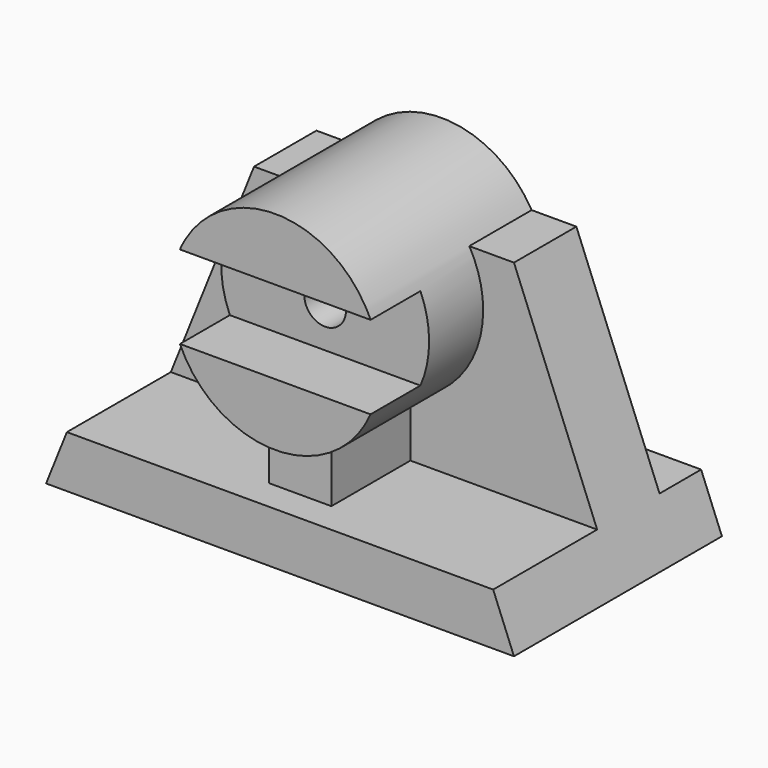
from build123d import *

# Parameters (mm, degrees)
F0_W      = 90
F0_H      = 50
F1_DEPTH  = 10
F2_W      = 90
F2_H      = 15
F3_DEPTH  = 40
F4_SIZE2  = 49.99999
F4_SIZE   = 19.99999
F5_SIZE2  = 19.99999
F5_SIZE   = 49.99999
F7_DEPTH  = 25
F8_DEPTH  = 15
F9_DEPTH  = 13
F10_DEPTH = 19
F11_R     = 4
F12_DEPTH = 40


# Not quite as in the source:
# - a fillet or chamfer is up to 0.001 mm smaller than in the source, because OpenCascade refuses the exact size


with BuildPart() as f1:
    # F0 (on Top) → F1 (new body)
    with BuildSketch(Plane.XY):
        with Locations((0.9217737243, 10.8652876893)):
            Rectangle(F0_W, F0_H)
    extrude(amount=F1_DEPTH)

    # F2 (on face) → F3 (join)
    with BuildSketch(Plane.XY.offset(10)):
        with Locations((0.9217737243, 18.3652876893)):
            Rectangle(F2_W, F2_H)
    extrude(amount=F3_DEPTH)

    # F4 (size 20 and 50 in the source; OpenCascade refuses exactly that, so slightly less here)
    f4_edges = [f1.edges().sort_by_distance(p)[0] for p in [
        (-44.078226, 18.365288, 50),
    ]]
    f4_side = f1.faces().sort_by_distance((0.921774, 18.365288, 50))[0]
    chamfer(f4_edges, length=F4_SIZE, length2=F4_SIZE2, reference=f4_side)

    # F5 (size 50 and 20 in the source; OpenCascade refuses exactly that, so slightly less here)
    f5_edges = [f1.edges().sort_by_distance(p)[0] for p in [
        (45.921774, 18.365288, 50),
    ]]
    f5_side = f1.faces().sort_by_distance((45.921774, 14.956197, 18.636364))[0]
    chamfer(f5_edges, length=F5_SIZE, length2=F5_SIZE2, reference=f5_side)

    # F6 (on face) → F7 (join)
    with BuildSketch(Plane.XZ.offset(-10.8652876893)):
        with BuildLine():
            Line((-17.3205080757, 50), (17.3205080757, 50))
            ThreePointArc((17.3205080757, 50), (0, 60), (-17.3205080757, 50))
        make_face()
        with BuildLine():
            Line((-18.3303027798, 48), (18.3303027798, 48))
            ThreePointArc((18.3303027798, 48), (17.8534332458, 49.0141511711), (17.3205080757, 50))
            Line((17.3205080757, 50), (-17.3205080757, 50))
            ThreePointArc((-17.3205080757, 50), (-17.8534332458, 49.0141511711), (-18.3303027798, 48))
        make_face()
        with BuildLine():
            ThreePointArc((6, 20.9212159717), (13.3669657075, 25.1230302893), (18.3303027798, 32))
            Line((18.3303027798, 32), (-18.3303027798, 32))
            ThreePointArc((-18.3303027798, 32), (-13.3669657075, 25.1230302893), (-6, 20.9212159717))
            ThreePointArc((-6, 20.9212159717), (0, 20), (6, 20.9212159717))
        make_face()
    extrude(amount=F7_DEPTH)

    # F8 (add): a face of the model
    f8_faces = [f1.faces().sort_by_distance(p)[0] for p in [
        (0, 10.8652876893, 54.100403238),
    ]]
    extrude(f8_faces, amount=F8_DEPTH)

    # F6 (on face) → F9 (join)
    with BuildSketch(Plane.XZ.offset(-10.8652876893)):
        with BuildLine():
            ThreePointArc((18.3303027798, 32), (19.5781262586, 35.9138071262), (20, 40))
            ThreePointArc((20, 40), (19.5781262586, 44.0861928738), (18.3303027798, 48))
            Line((18.3303027798, 48), (-18.3303027798, 48))
            ThreePointArc((-18.3303027798, 48), (-20, 40), (-18.3303027798, 32))
            Line((-18.3303027798, 32), (18.3303027798, 32))
        make_face()
    extrude(amount=F9_DEPTH)

    # F6 (on face) → F10 (join)
    with BuildSketch(Plane.XZ.offset(-10.8652876893)):
        with BuildLine():
            Line((6, 10), (6, 20.9212159717))
            ThreePointArc((6, 20.9212159717), (0, 20), (-6, 20.9212159717))
            Line((-6, 20.9212159717), (-6, 10))
            Line((-6, 10), (6, 10))
        make_face()
    extrude(amount=F10_DEPTH)

    # F11 (on face) → F12 (cut)
    with BuildSketch(Plane.XZ.offset(2.1347123107)):
        with Locations((0, 40)):
            Circle(F11_R)
    extrude(amount=-F12_DEPTH, mode=Mode.SUBTRACT)


solid = f1.part
